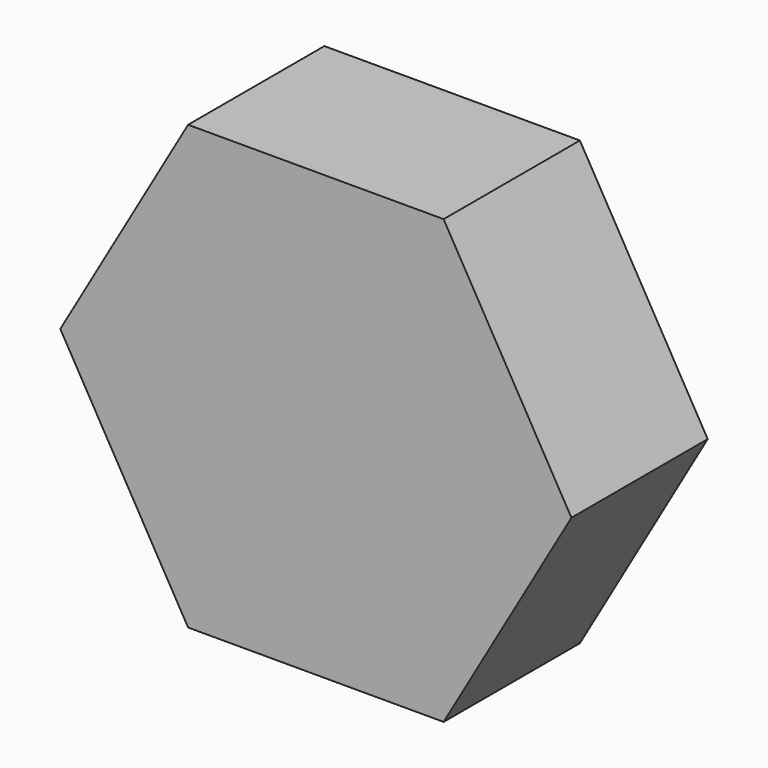
from build123d import *

# Parameters (mm, degrees)
F1_DEPTH = 6.35


# Not quite as in the source:
# - the program builds the solid bodies; features that only make, move or delete a surface that nothing else refers to are left out


with BuildPart() as f1:
    # F0 (on Front) → F1 (new body)
    with BuildSketch(Plane.XZ):
        Polygon((-4.7625, -8.248891971), (4.7625, -8.248891971), (9.525, 0), (4.7625, 8.248891971), (-4.7625, 8.248891971), (-9.525, 0), align=None)
    extrude(amount=F1_DEPTH)


solid = f1.part
